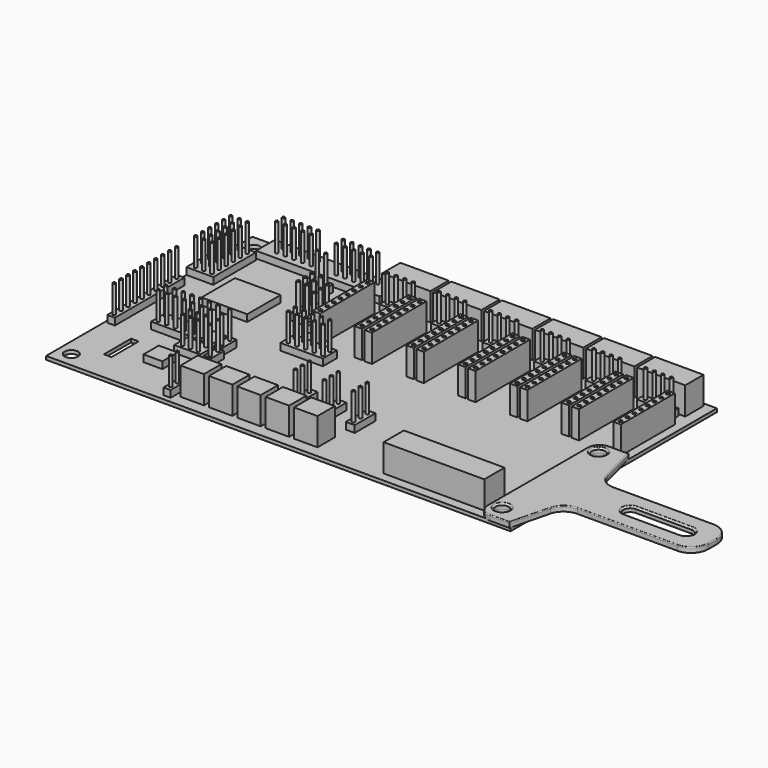
from build123d import *

# Parameters (mm, degrees)
F0_W           = 2.1383463393
F0_H           = 19.7797067453
F0_R           = 0.4865075134
F1_DEPTH       = 8
F0_H_2         = 19.6269687937
F0_R_2         = 1.9460300534
F0_W_2         = 2.2147138911
F0_H_3         = 9.8727391815
F0_W_3         = 5.479511394
F0_H_4         = 5.554471502
F0_W_4         = 2.0619777519
F0_H_5         = 4.9640203219
F0_W_5         = 6.8159792801
F0_H_6         = 6.2813939898
F0_W_6         = 2.5666546012
F0_H_7         = 7.4842127053
F0_W_7         = 7.560583364
F0_H_8         = 4.8876486276
F0_W_8         = 2.1383453036
F0_H_9         = 4.6859326135
F0_W_9         = 17.6604543653
F0_H_10        = 5.1752777491
F0_W_10        = 2.2910845498
F0_H_11        = 25.2068089793
F0_W_11        = 13.2490306353
F0_H_12        = 12.1427537582
F0_W_12        = 12.365488222
F0_H_13        = 5.121120681
F0_W_13        = 2.2910866211
F0_H_14        = 7.1787352486
F0_W_14        = 5.0641262077
F0_H_15        = 7.3660017566
F0_W_15        = 4.9640203219
F0_H_16        = 2.4147640345
F0_R_3         = 1.6205905882
F0_W_16        = 10.0807783365
F0_H_17        = 2.5201944547
F0_W_17        = 14.0519930406
F0_H_18        = 6.6441499584
F2_DEPTH       = 1
F0_W_18        = 7.8297872952
F0_H_19        = 15.5030138078
F0_R_4         = 0.41700644
F0_W_19        = 17.9754786721
F0_H_20        = 6.8159803158
F3_DEPTH       = 2
F3_DEPTH_BACK  = 1
F0_W_20        = 9.8887440656
F0_H_21        = 7.3633516746
F0_W_21        = 9.622558009
F0_W_22        = 9.7573204997
F4_DEPTH       = 8
F4_DEPTH_BACK  = 1
F0_R_5         = 0.5
F5_DEPTH       = 2
F5_DEPTH_BACK  = 1
F6_DEPTH       = 8
F6_DEPTH_BACK  = 1
F7_DEPTH       = 2
F7_DEPTH_BACK  = 1
F8_R           = 2.1799728678
F8_R_2         = 2
F8_R_3         = 2.5
F9_DEPTH       = 4
F10_DEPTH      = 10
F10_DEPTH_BACK = 1
F11_R          = 1.9460300534
F12_DEPTH      = 1.5
F13_SIZE       = 0.5
F14_R          = 0.25


# Not quite as in the source:
# - a feature names something its author has since deleted; it is built from what else it names


with BuildPart() as f1:
    # F0 (on Top) → F1 (new body)
    with BuildSketch(Plane.XY):
        with Locations((5.3948195173, 11.5601837436)):
            Rectangle(F0_W, F0_H)
        with Locations((5.4469605535, 3.0105938525)):
            Circle(F0_R, mode=Mode.SUBTRACT)
        with Locations((5.439511834, 5.4706814883)):
            Circle(F0_R, mode=Mode.SUBTRACT)
        with Locations((5.4320631146, 7.9307691241)):
            Circle(F0_R, mode=Mode.SUBTRACT)
        with Locations((5.4246143951, 10.3908567598)):
            Circle(F0_R, mode=Mode.SUBTRACT)
        with Locations((5.4171656757, 12.8509443956)):
            Circle(F0_R, mode=Mode.SUBTRACT)
        with Locations((5.4097169562, 15.3110320313)):
            Circle(F0_R, mode=Mode.SUBTRACT)
        with Locations((5.4022682368, 17.7711196671)):
            Circle(F0_R, mode=Mode.SUBTRACT)
        with Locations((5.3948195173, 20.2312073029)):
            Circle(F0_R, mode=Mode.SUBTRACT)
    extrude(amount=F1_DEPTH)

    # F8 (on face) → F9 (cut)
    with BuildSketch(Plane.XY.offset(8)):
        with Locations((-23.1175161898, -59.319212369)):
            Circle(F8_R)
        with Locations((-16.9533622074, -59.319212369)):
            Circle(F8_R_2)
        with Locations((-8.2318261898, -59.319212369)):
            Circle(F8_R)
        with Locations((-2.0676722074, -59.319212369)):
            Circle(F8_R_2)
        with Locations((6.6538638102, -59.319212369)):
            Circle(F8_R)
        with Locations((12.8180177926, -59.319212369)):
            Circle(F8_R_2)
        with Locations((21.5395538102, -59.319212369)):
            Circle(F8_R)
        with Locations((27.7037077926, -59.319212369)):
            Circle(F8_R_2)
        with Locations((36.4252438102, -59.319212369)):
            Circle(F8_R)
        with Locations((42.5893977926, -59.319212369)):
            Circle(F8_R_2)
        with Locations((84.719479084, -59.7627162933)):
            Circle(F8_R_3)
        with Locations((93.9138680696, -59.7627162933)):
            Circle(F8_R_3)
        with Locations((102.625829084, -59.7627162933)):
            Circle(F8_R_3)
        with Locations((111.8202180696, -59.7627162933)):
            Circle(F8_R_3)
        with Locations((120.532179084, -59.7627162933)):
            Circle(F8_R_3)
        with Locations((129.7265680696, -59.7627162933)):
            Circle(F8_R_3)
    extrude(amount=-F9_DEPTH, mode=Mode.SUBTRACT)


with BuildPart() as f1b:
    # F0 (on Top) → F1, piece 2 (new body)
    with BuildSketch(Plane.XY):
        with Locations((17.4835866574, 11.560184132)):
            Rectangle(F0_W, F0_H_2)
        with Locations((17.538712812, 3.0105938525)):
            Circle(F0_R, mode=Mode.SUBTRACT)
        with Locations((17.5312640925, 5.4706814883)):
            Circle(F0_R, mode=Mode.SUBTRACT)
        with Locations((17.5238153731, 7.9307691241)):
            Circle(F0_R, mode=Mode.SUBTRACT)
        with Locations((17.5163666537, 10.3908567598)):
            Circle(F0_R, mode=Mode.SUBTRACT)
        with Locations((17.5089179342, 12.8509443956)):
            Circle(F0_R, mode=Mode.SUBTRACT)
        with Locations((17.5014692148, 15.3110320313)):
            Circle(F0_R, mode=Mode.SUBTRACT)
        with Locations((17.4940204953, 17.7711196671)):
            Circle(F0_R, mode=Mode.SUBTRACT)
        with Locations((17.4865717759, 20.2312073029)):
            Circle(F0_R, mode=Mode.SUBTRACT)
    extrude(amount=F1_DEPTH)


with BuildPart() as f1c:
    # F0 (on Top) → F1, piece 3 (new body)
    with BuildSketch(Plane.XY):
        with Locations((20.4430973949, 11.5601837436)):
            Rectangle(F0_W, F0_H)
        with Locations((20.4900175104, 3.0105938525)):
            Circle(F0_R, mode=Mode.SUBTRACT)
        with Locations((20.4825687909, 5.4706814883)):
            Circle(F0_R, mode=Mode.SUBTRACT)
        with Locations((20.4751200715, 7.9307691241)):
            Circle(F0_R, mode=Mode.SUBTRACT)
        with Locations((20.467671352, 10.3908567598)):
            Circle(F0_R, mode=Mode.SUBTRACT)
        with Locations((20.4602226326, 12.8509443956)):
            Circle(F0_R, mode=Mode.SUBTRACT)
        with Locations((20.4527739131, 15.3110320313)):
            Circle(F0_R, mode=Mode.SUBTRACT)
        with Locations((20.4453251937, 17.7711196671)):
            Circle(F0_R, mode=Mode.SUBTRACT)
        with Locations((20.4378764742, 20.2312073029)):
            Circle(F0_R, mode=Mode.SUBTRACT)
    extrude(amount=F1_DEPTH)


with BuildPart() as f1d:
    # F0 (on Top) → F1, piece 4 (new body)
    with BuildSketch(Plane.XY):
        with Locations((32.5318645349, 11.560184132)):
            Rectangle(F0_W, F0_H_2)
        with Locations((32.5817697689, 3.0105938525)):
            Circle(F0_R, mode=Mode.SUBTRACT)
        with Locations((32.5743210495, 5.4706814883)):
            Circle(F0_R, mode=Mode.SUBTRACT)
        with Locations((32.56687233, 7.9307691241)):
            Circle(F0_R, mode=Mode.SUBTRACT)
        with Locations((32.5594236106, 10.3908567598)):
            Circle(F0_R, mode=Mode.SUBTRACT)
        with Locations((32.5519748911, 12.8509443956)):
            Circle(F0_R, mode=Mode.SUBTRACT)
        with Locations((32.5445261717, 15.3110320313)):
            Circle(F0_R, mode=Mode.SUBTRACT)
        with Locations((32.5370774522, 17.7711196671)):
            Circle(F0_R, mode=Mode.SUBTRACT)
        with Locations((32.5296287328, 20.2312073029)):
            Circle(F0_R, mode=Mode.SUBTRACT)
    extrude(amount=F1_DEPTH)


with BuildPart() as f1e:
    # F0 (on Top) → F1, piece 5 (new body)
    with BuildSketch(Plane.XY):
        with Locations((35.4913752724, 11.5601837436)):
            Rectangle(F0_W, F0_H)
        with Locations((35.5330744673, 3.0105938525)):
            Circle(F0_R, mode=Mode.SUBTRACT)
        with Locations((35.5256257478, 5.4706814883)):
            Circle(F0_R, mode=Mode.SUBTRACT)
        with Locations((35.5181770284, 7.9307691241)):
            Circle(F0_R, mode=Mode.SUBTRACT)
        with Locations((35.5107283089, 10.3908567598)):
            Circle(F0_R, mode=Mode.SUBTRACT)
        with Locations((35.5032795895, 12.8509443956)):
            Circle(F0_R, mode=Mode.SUBTRACT)
        with Locations((35.49583087, 15.3110320313)):
            Circle(F0_R, mode=Mode.SUBTRACT)
        with Locations((35.4883821506, 17.7711196671)):
            Circle(F0_R, mode=Mode.SUBTRACT)
        with Locations((35.4809334311, 20.2312073029)):
            Circle(F0_R, mode=Mode.SUBTRACT)
    extrude(amount=F1_DEPTH)


with BuildPart() as f1f:
    # F0 (on Top) → F1, piece 6 (new body)
    with BuildSketch(Plane.XY):
        with Locations((47.5801424125, 11.560184132)):
            Rectangle(F0_W, F0_H_2)
        with Locations((47.6248267258, 3.0105938525)):
            Circle(F0_R, mode=Mode.SUBTRACT)
        with Locations((47.6173780064, 5.4706814883)):
            Circle(F0_R, mode=Mode.SUBTRACT)
        with Locations((47.6099292869, 7.9307691241)):
            Circle(F0_R, mode=Mode.SUBTRACT)
        with Locations((47.6024805675, 10.3908567598)):
            Circle(F0_R, mode=Mode.SUBTRACT)
        with Locations((47.595031848, 12.8509443956)):
            Circle(F0_R, mode=Mode.SUBTRACT)
        with Locations((47.5875831286, 15.3110320313)):
            Circle(F0_R, mode=Mode.SUBTRACT)
        with Locations((47.5801344091, 17.7711196671)):
            Circle(F0_R, mode=Mode.SUBTRACT)
        with Locations((47.5726856897, 20.2312073029)):
            Circle(F0_R, mode=Mode.SUBTRACT)
    extrude(amount=F1_DEPTH)


with BuildPart() as f1g:
    # F0 (on Top) → F1, piece 7 (new body)
    with BuildSketch(Plane.XY):
        with Locations((50.5396531499, 11.5601837436)):
            Rectangle(F0_W, F0_H)
        with Locations((50.5761314242, 3.0105938525)):
            Circle(F0_R, mode=Mode.SUBTRACT)
        with Locations((50.5686827047, 5.4706814883)):
            Circle(F0_R, mode=Mode.SUBTRACT)
        with Locations((50.5612339853, 7.9307691241)):
            Circle(F0_R, mode=Mode.SUBTRACT)
        with Locations((50.5537852658, 10.3908567598)):
            Circle(F0_R, mode=Mode.SUBTRACT)
        with Locations((50.5463365464, 12.8509443956)):
            Circle(F0_R, mode=Mode.SUBTRACT)
        with Locations((50.5388878269, 15.3110320313)):
            Circle(F0_R, mode=Mode.SUBTRACT)
        with Locations((50.5314391075, 17.7711196671)):
            Circle(F0_R, mode=Mode.SUBTRACT)
        with Locations((50.523990388, 20.2312073029)):
            Circle(F0_R, mode=Mode.SUBTRACT)
    extrude(amount=F1_DEPTH)


with BuildPart() as f1h:
    # F0 (on Top) → F1, piece 8 (new body)
    with BuildSketch(Plane.XY):
        with Locations((62.62842029, 11.560184132)):
            Rectangle(F0_W, F0_H_2)
        with Locations((62.6678836827, 3.0105938525)):
            Circle(F0_R, mode=Mode.SUBTRACT)
        with Locations((62.6604349633, 5.4706814883)):
            Circle(F0_R, mode=Mode.SUBTRACT)
        with Locations((62.6529862438, 7.9307691241)):
            Circle(F0_R, mode=Mode.SUBTRACT)
        with Locations((62.6455375244, 10.3908567598)):
            Circle(F0_R, mode=Mode.SUBTRACT)
        with Locations((62.6380888049, 12.8509443956)):
            Circle(F0_R, mode=Mode.SUBTRACT)
        with Locations((62.6306400855, 15.3110320313)):
            Circle(F0_R, mode=Mode.SUBTRACT)
        with Locations((62.623191366, 17.7711196671)):
            Circle(F0_R, mode=Mode.SUBTRACT)
        with Locations((62.6157426466, 20.2312073029)):
            Circle(F0_R, mode=Mode.SUBTRACT)
    extrude(amount=F1_DEPTH)


with BuildPart() as f1i:
    # F0 (on Top) → F1, piece 9 (new body)
    with BuildSketch(Plane.XY):
        with Locations((65.5879310275, 11.5601837436)):
            Rectangle(F0_W, F0_H)
        with Locations((65.6191883811, 3.0105938525)):
            Circle(F0_R, mode=Mode.SUBTRACT)
        with Locations((65.6117396616, 5.4706814883)):
            Circle(F0_R, mode=Mode.SUBTRACT)
        with Locations((65.6042909422, 7.9307691241)):
            Circle(F0_R, mode=Mode.SUBTRACT)
        with Locations((65.5968422228, 10.3908567598)):
            Circle(F0_R, mode=Mode.SUBTRACT)
        with Locations((65.5893935033, 12.8509443956)):
            Circle(F0_R, mode=Mode.SUBTRACT)
        with Locations((65.5819447839, 15.3110320313)):
            Circle(F0_R, mode=Mode.SUBTRACT)
        with Locations((65.5744960644, 17.7711196671)):
            Circle(F0_R, mode=Mode.SUBTRACT)
        with Locations((65.567047345, 20.2312073029)):
            Circle(F0_R, mode=Mode.SUBTRACT)
    extrude(amount=F1_DEPTH)


with BuildPart() as f1j:
    # F0 (on Top) → F1, piece 10 (new body)
    with BuildSketch(Plane.XY):
        with Locations((77.6766981675, 11.560184132)):
            Rectangle(F0_W, F0_H_2)
        with Locations((77.7109406396, 3.0105938525)):
            Circle(F0_R, mode=Mode.SUBTRACT)
        with Locations((77.7034919202, 5.4706814883)):
            Circle(F0_R, mode=Mode.SUBTRACT)
        with Locations((77.6960432007, 7.9307691241)):
            Circle(F0_R, mode=Mode.SUBTRACT)
        with Locations((77.6885944813, 10.3908567598)):
            Circle(F0_R, mode=Mode.SUBTRACT)
        with Locations((77.6811457618, 12.8509443956)):
            Circle(F0_R, mode=Mode.SUBTRACT)
        with Locations((77.6736970424, 15.3110320313)):
            Circle(F0_R, mode=Mode.SUBTRACT)
        with Locations((77.6662483229, 17.7711196671)):
            Circle(F0_R, mode=Mode.SUBTRACT)
        with Locations((77.6587996035, 20.2312073029)):
            Circle(F0_R, mode=Mode.SUBTRACT)
    extrude(amount=F1_DEPTH)


with BuildPart() as f1k:
    # F0 (on Top) → F1, piece 11 (new body)
    with BuildSketch(Plane.XY):
        with Locations((80.636208905, 11.5601837436)):
            Rectangle(F0_W, F0_H)
        with Locations((80.662245338, 3.0105938525)):
            Circle(F0_R, mode=Mode.SUBTRACT)
        with Locations((80.6547966186, 5.4706814883)):
            Circle(F0_R, mode=Mode.SUBTRACT)
        with Locations((80.6473478991, 7.9307691241)):
            Circle(F0_R, mode=Mode.SUBTRACT)
        with Locations((80.6398991797, 10.3908567598)):
            Circle(F0_R, mode=Mode.SUBTRACT)
        with Locations((80.6324504602, 12.8509443956)):
            Circle(F0_R, mode=Mode.SUBTRACT)
        with Locations((80.6250017408, 15.3110320313)):
            Circle(F0_R, mode=Mode.SUBTRACT)
        with Locations((80.6175530213, 17.7711196671)):
            Circle(F0_R, mode=Mode.SUBTRACT)
        with Locations((80.6101043019, 20.2312073029)):
            Circle(F0_R, mode=Mode.SUBTRACT)
    extrude(amount=F1_DEPTH)


with BuildPart() as f1l:
    # F0 (on Top) → F1, piece 12 (new body)
    with BuildSketch(Plane.XY):
        with Locations((92.7249760451, 11.560184132)):
            Rectangle(F0_W, F0_H_2)
        with Locations((92.7539975965, 3.0105938525)):
            Circle(F0_R, mode=Mode.SUBTRACT)
        with Locations((92.7465488771, 5.4706814883)):
            Circle(F0_R, mode=Mode.SUBTRACT)
        with Locations((92.7391001577, 7.9307691241)):
            Circle(F0_R, mode=Mode.SUBTRACT)
        with Locations((92.7316514382, 10.3908567598)):
            Circle(F0_R, mode=Mode.SUBTRACT)
        with Locations((92.7242027188, 12.8509443956)):
            Circle(F0_R, mode=Mode.SUBTRACT)
        with Locations((92.7167539993, 15.3110320313)):
            Circle(F0_R, mode=Mode.SUBTRACT)
        with Locations((92.7093052799, 17.7711196671)):
            Circle(F0_R, mode=Mode.SUBTRACT)
        with Locations((92.7018565604, 20.2312073029)):
            Circle(F0_R, mode=Mode.SUBTRACT)
    extrude(amount=F1_DEPTH)


with BuildPart() as f2:
    # F0 (on Top) → F2 (new body)
    with BuildSketch(Plane.XY):
        Polygon((-38.7532671023, 33.5722392425), (-38.7532671023, 31.7772014981), (-38.7532671023, 25.0439776386), (-30.9234798072, 25.0439776386), (-30.9234798072, 9.5409638307), (-38.7532671023, 9.5409638307), (-38.7532671023, -41.4277607575), (96.2467328977, -41.4277607575), (96.2467328977, 33.5722392425), align=None)
        with Locations((-34.8440401784, -37.1435576593)):
            Circle(F0_R_2, mode=Mode.SUBTRACT)
        with Locations((-27.887346881, -27.6786446647)):
            Rectangle(F0_W_2, F0_H_3, mode=Mode.SUBTRACT)
        with Locations((-16.8053327625, -27.2508614757)):
            Rectangle(F0_W_3, F0_H_4, mode=Mode.SUBTRACT)
        with Locations((-4.8237512626, -37.3881089662)):
            Rectangle(F0_W_4, F0_H_5, mode=Mode.SUBTRACT)
        with Locations((1.0400285531, -34.9124877097)):
            Rectangle(F0_W_5, F0_H_6, mode=Mode.SUBTRACT)
        with Locations((9.2893166707, -34.9124877097)):
            Rectangle(F0_W_5, F0_H_6, mode=Mode.SUBTRACT)
        with Locations((17.5386047883, -34.9124877097)):
            Rectangle(F0_W_5, F0_H_6, mode=Mode.SUBTRACT)
        with Locations((25.7878929059, -34.9124877097)):
            Rectangle(F0_W_5, F0_H_6, mode=Mode.SUBTRACT)
        with Locations((21.5385374591, -23.5010766555)):
            Rectangle(F0_W_6, F0_H_7, mode=Mode.SUBTRACT)
        with Locations((-13.2243989271, -19.6321943845)):
            Rectangle(F0_W_7, F0_H_8, mode=Mode.SUBTRACT)
        with Locations((-7.3821305288, -19.6554254934)):
            Rectangle(F0_W_8, F0_H_9, mode=Mode.SUBTRACT)
        with Locations((-19.4389688494, -13.7994720597)):
            Rectangle(F0_W_9, F0_H_10, mode=Mode.SUBTRACT)
        with Locations((-8.7009054267, -13.773147992)):
            Rectangle(F0_W_10, F0_H_10, mode=Mode.SUBTRACT)
        with Locations((-36.9753206354, -7.4155029606)):
            Rectangle(F0_W_2, F0_H_11, mode=Mode.SUBTRACT)
        with Locations((34.0371810235, -34.9124877097)):
            Rectangle(F0_W_5, F0_H_6, mode=Mode.SUBTRACT)
        with Locations((29.940144129, -23.5010766555)):
            Rectangle(F0_W_6, F0_H_7, mode=Mode.SUBTRACT)
        with Locations((38.3417507989, -23.5010766555)):
            Rectangle(F0_W_6, F0_H_7, mode=Mode.SUBTRACT)
        Polygon((57.1692081971, -38.6863915229), (57.1692081971, -31.3230398483), (67.0579522627, -31.3230398483), (76.6805102716, -31.3230398483), (86.4378307714, -31.3230398483), (86.4378307714, -38.6863915229), (76.6805102716, -38.6863915229), (67.0579522627, -38.6863915229), align=None, mode=Mode.SUBTRACT)
        with Locations((90.3885619373, -37.1455874826)):
            Circle(F0_R_2, mode=Mode.SUBTRACT)
        with Locations((-20.1162074077, 6.1425196168)):
            Rectangle(F0_W_11, F0_H_12, mode=Mode.SUBTRACT)
        with Locations((7.3327940732, -3.6349598129)):
            Rectangle(F0_W_12, F0_H_13, mode=Mode.SUBTRACT)
        with Locations((1.1712568996, 8.2426817919)):
            Rectangle(F0_W_13, F0_H_14, mode=Mode.SUBTRACT)
        with Locations((-3.7398368359, 10.5292772493)):
            Rectangle(F0_W_14, F0_H_15, mode=Mode.SUBTRACT)
        with Locations((5.3948195173, 11.5601837436)):
            Rectangle(F0_W, F0_H, mode=Mode.SUBTRACT)
        with Locations((17.4835866574, 11.560184132)):
            Rectangle(F0_W, F0_H_2, mode=Mode.SUBTRACT)
        with Locations((20.4430973949, 11.5601837436)):
            Rectangle(F0_W, F0_H, mode=Mode.SUBTRACT)
        with Locations((-9.9405092772, 22.5856218906)):
            Rectangle(F0_W_15, F0_H_16, mode=Mode.SUBTRACT)
        with Locations((-34.9667365808, 29.4120077307)):
            Circle(F0_R_3, mode=Mode.SUBTRACT)
        Polygon((-31.4407066232, 25.7186289664), (-31.4407066232, 32.5346092821), (-13.4652279511, 32.5346092821), (4.510250721, 32.5346092821), (4.510250721, 25.7186289664), (-13.4652279511, 25.7186289664), align=None, mode=Mode.SUBTRACT)
        with Locations((11.9188682081, 23.9329783236)):
            Rectangle(F0_W_16, F0_H_17, mode=Mode.SUBTRACT)
        with Locations((26.8882540273, 23.9329783236)):
            Rectangle(F0_W_16, F0_H_17, mode=Mode.SUBTRACT)
        with Locations((12.0708325316, 29.2316274854)):
            Rectangle(F0_W_17, F0_H_18, mode=Mode.SUBTRACT)
        with Locations((26.887482792, 29.2316274854)):
            Rectangle(F0_W_17, F0_H_18, mode=Mode.SUBTRACT)
        with Locations((32.5318645349, 11.560184132)):
            Rectangle(F0_W, F0_H_2, mode=Mode.SUBTRACT)
        with Locations((35.4913752724, 11.5601837436)):
            Rectangle(F0_W, F0_H, mode=Mode.SUBTRACT)
        with Locations((47.5801424125, 11.560184132)):
            Rectangle(F0_W, F0_H_2, mode=Mode.SUBTRACT)
        with Locations((50.5396531499, 11.5601837436)):
            Rectangle(F0_W, F0_H, mode=Mode.SUBTRACT)
        with Locations((90.3885619373, -2.1260819313)):
            Circle(F0_R_2, mode=Mode.SUBTRACT)
        with Locations((62.62842029, 11.560184132)):
            Rectangle(F0_W, F0_H_2, mode=Mode.SUBTRACT)
        with Locations((65.5879310275, 11.5601837436)):
            Rectangle(F0_W, F0_H, mode=Mode.SUBTRACT)
        with Locations((77.6766981675, 11.560184132)):
            Rectangle(F0_W, F0_H_2, mode=Mode.SUBTRACT)
        with Locations((80.636208905, 11.5601837436)):
            Rectangle(F0_W, F0_H, mode=Mode.SUBTRACT)
        with Locations((92.7249760451, 11.560184132)):
            Rectangle(F0_W, F0_H_2, mode=Mode.SUBTRACT)
        with Locations((41.8576398464, 23.9329783236)):
            Rectangle(F0_W_16, F0_H_17, mode=Mode.SUBTRACT)
        with Locations((56.8270256656, 23.9329783236)):
            Rectangle(F0_W_16, F0_H_17, mode=Mode.SUBTRACT)
        with Locations((41.7041330524, 29.2316274854)):
            Rectangle(F0_W_17, F0_H_18, mode=Mode.SUBTRACT)
        with Locations((56.5207833128, 29.2316274854)):
            Rectangle(F0_W_17, F0_H_18, mode=Mode.SUBTRACT)
        with Locations((71.7964114848, 23.9329783236)):
            Rectangle(F0_W_16, F0_H_17, mode=Mode.SUBTRACT)
        with Locations((86.765797304, 23.9329783236)):
            Rectangle(F0_W_16, F0_H_17, mode=Mode.SUBTRACT)
        with Locations((71.3374335732, 29.2316274854)):
            Rectangle(F0_W_17, F0_H_18, mode=Mode.SUBTRACT)
        with Locations((86.1540838336, 29.2316274854)):
            Rectangle(F0_W_17, F0_H_18, mode=Mode.SUBTRACT)
    extrude(amount=-F2_DEPTH)

    # F0 (on Top) → F3 (join, two sides)
    with BuildSketch(Plane.XY) as f3_sk:
        with Locations((-34.8383734548, 17.2924707347)):
            Rectangle(F0_W_18, F0_H_19)
        with Locations((-37.078142586, 10.8069347614)):
            Circle(F0_R_4, mode=Mode.SUBTRACT)
        with Locations((-34.6817455773, 10.8069347614)):
            Circle(F0_R_4, mode=Mode.SUBTRACT)
        with Locations((-32.2853485686, 10.8069347614)):
            Circle(F0_R_4, mode=Mode.SUBTRACT)
        with Locations((-37.0635132799, 13.3533761215)):
            Circle(F0_R_4, mode=Mode.SUBTRACT)
        with Locations((-34.6671162713, 13.3533761215)):
            Circle(F0_R_4, mode=Mode.SUBTRACT)
        with Locations((-32.2707192626, 13.3533761215)):
            Circle(F0_R_4, mode=Mode.SUBTRACT)
        with Locations((-37.0488839739, 15.8998174816)):
            Circle(F0_R_4, mode=Mode.SUBTRACT)
        with Locations((-34.6524869652, 15.8998174816)):
            Circle(F0_R_4, mode=Mode.SUBTRACT)
        with Locations((-32.2560899566, 15.8998174816)):
            Circle(F0_R_4, mode=Mode.SUBTRACT)
        with Locations((-37.0342546679, 18.4462588418)):
            Circle(F0_R_4, mode=Mode.SUBTRACT)
        with Locations((-34.6378576592, 18.4462588418)):
            Circle(F0_R_4, mode=Mode.SUBTRACT)
        with Locations((-32.2414606505, 18.4462588418)):
            Circle(F0_R_4, mode=Mode.SUBTRACT)
        with Locations((-37.0196253619, 20.9927002019)):
            Circle(F0_R_4, mode=Mode.SUBTRACT)
        with Locations((-34.6232283532, 20.9927002019)):
            Circle(F0_R_4, mode=Mode.SUBTRACT)
        with Locations((-32.2268313445, 20.9927002019)):
            Circle(F0_R_4, mode=Mode.SUBTRACT)
        with Locations((-37.0049960558, 23.5391415621)):
            Circle(F0_R_4, mode=Mode.SUBTRACT)
        with Locations((-34.6085990472, 23.5391415621)):
            Circle(F0_R_4, mode=Mode.SUBTRACT)
        with Locations((-32.2122020385, 23.5391415621)):
            Circle(F0_R_4, mode=Mode.SUBTRACT)
        with Locations((-19.4389688494, -13.7994720597)):
            Rectangle(F0_W_9, F0_H_10)
        with Locations((-27.1577291654, -15.2034537075)):
            Circle(F0_R_4, mode=Mode.SUBTRACT)
        with Locations((-24.6314429908, -15.2034537075)):
            Circle(F0_R_4, mode=Mode.SUBTRACT)
        with Locations((-22.1051568161, -15.2034537075)):
            Circle(F0_R_4, mode=Mode.SUBTRACT)
        with Locations((-19.5788706415, -15.2034537075)):
            Circle(F0_R_4, mode=Mode.SUBTRACT)
        with Locations((-17.0525844669, -15.2034537075)):
            Circle(F0_R_4, mode=Mode.SUBTRACT)
        with Locations((-14.5262982923, -15.2034537075)):
            Circle(F0_R_4, mode=Mode.SUBTRACT)
        with Locations((-12.0000121177, -15.2034537075)):
            Circle(F0_R_4, mode=Mode.SUBTRACT)
        with Locations((-27.1577291654, -12.3954904119)):
            Circle(F0_R_4, mode=Mode.SUBTRACT)
        with Locations((-24.6314429908, -12.3954904119)):
            Circle(F0_R_4, mode=Mode.SUBTRACT)
        with Locations((-22.1051568161, -12.3954904119)):
            Circle(F0_R_4, mode=Mode.SUBTRACT)
        with Locations((-19.5788706415, -12.3954904119)):
            Circle(F0_R_4, mode=Mode.SUBTRACT)
        with Locations((-17.0525844669, -12.3954904119)):
            Circle(F0_R_4, mode=Mode.SUBTRACT)
        with Locations((-14.5262982923, -12.3954904119)):
            Circle(F0_R_4, mode=Mode.SUBTRACT)
        with Locations((-12.0000121177, -12.3954904119)):
            Circle(F0_R_4, mode=Mode.SUBTRACT)
        with Locations((-36.9753206354, -7.4155029606)):
            Rectangle(F0_W_2, F0_H_11)
        with Locations((-37.0629606711, -18.8174451744)):
            Circle(F0_R_4, mode=Mode.SUBTRACT)
        with Locations((-37.0629606711, -16.2902419244)):
            Circle(F0_R_4, mode=Mode.SUBTRACT)
        with Locations((-37.0629606711, -13.7630386744)):
            Circle(F0_R_4, mode=Mode.SUBTRACT)
        with Locations((-37.0629606711, -11.2358354244)):
            Circle(F0_R_4, mode=Mode.SUBTRACT)
        with Locations((-37.0629606711, -8.7086321744)):
            Circle(F0_R_4, mode=Mode.SUBTRACT)
        with Locations((-37.0629606711, -6.1814289244)):
            Circle(F0_R_4, mode=Mode.SUBTRACT)
        with Locations((-37.0629606711, -3.6542256744)):
            Circle(F0_R_4, mode=Mode.SUBTRACT)
        with Locations((-37.0629606711, -1.1270224244)):
            Circle(F0_R_4, mode=Mode.SUBTRACT)
        with Locations((-37.0629606711, 1.4001808255)):
            Circle(F0_R_4, mode=Mode.SUBTRACT)
        with Locations((-37.0629606711, 3.9273840755)):
            Circle(F0_R_4, mode=Mode.SUBTRACT)
        with Locations((7.3327940732, -3.6349598129)):
            Rectangle(F0_W_12, F0_H_13)
        with Locations((2.4687983345, -4.8963822812)):
            Circle(F0_R_4, mode=Mode.SUBTRACT)
        with Locations((4.9796886313, -4.8963822812)):
            Circle(F0_R_4, mode=Mode.SUBTRACT)
        with Locations((7.4905789281, -4.8963822812)):
            Circle(F0_R_4, mode=Mode.SUBTRACT)
        with Locations((10.001469225, -4.8963822812)):
            Circle(F0_R_4, mode=Mode.SUBTRACT)
        with Locations((12.5123595218, -4.8963822812)):
            Circle(F0_R_4, mode=Mode.SUBTRACT)
        with Locations((2.4687983345, -2.3735373447)):
            Circle(F0_R_4, mode=Mode.SUBTRACT)
        with Locations((4.9796886313, -2.3735373447)):
            Circle(F0_R_4, mode=Mode.SUBTRACT)
        with Locations((7.4905789281, -2.3735373447)):
            Circle(F0_R_4, mode=Mode.SUBTRACT)
        with Locations((10.001469225, -2.3735373447)):
            Circle(F0_R_4, mode=Mode.SUBTRACT)
        with Locations((12.5123595218, -2.3735373447)):
            Circle(F0_R_4, mode=Mode.SUBTRACT)
        with Locations((-4.477488615, 29.1266191242)):
            Rectangle(F0_W_19, F0_H_20)
        with Locations((-9.8162656838, 27.8998053443)):
            Circle(F0_R_4, mode=Mode.SUBTRACT)
        with Locations((-7.305380947, 27.8998053443)):
            Circle(F0_R_4, mode=Mode.SUBTRACT)
        with Locations((-9.8162656838, 30.3534329042)):
            Circle(F0_R_4, mode=Mode.SUBTRACT)
        with Locations((-7.305380947, 30.3534329042)):
            Circle(F0_R_4, mode=Mode.SUBTRACT)
        with Locations((-4.7944962103, 27.8998053443)):
            Circle(F0_R_4, mode=Mode.SUBTRACT)
        with Locations((-2.2836114735, 27.8998053443)):
            Circle(F0_R_4, mode=Mode.SUBTRACT)
        with Locations((0.2272732632, 27.8998053443)):
            Circle(F0_R_4, mode=Mode.SUBTRACT)
        with Locations((-4.7944962103, 30.3534329042)):
            Circle(F0_R_4, mode=Mode.SUBTRACT)
        with Locations((-2.2836114735, 30.3534329042)):
            Circle(F0_R_4, mode=Mode.SUBTRACT)
        with Locations((0.2272732632, 30.3534329042)):
            Circle(F0_R_4, mode=Mode.SUBTRACT)
        with Locations((-22.4529672871, 29.1266191242)):
            Rectangle(F0_W_19, F0_H_20)
        with Locations((-27.1577291654, 27.8998053443)):
            Circle(F0_R_4, mode=Mode.SUBTRACT)
        with Locations((-24.6468444286, 27.8998053443)):
            Circle(F0_R_4, mode=Mode.SUBTRACT)
        with Locations((-22.1359596919, 27.8998053443)):
            Circle(F0_R_4, mode=Mode.SUBTRACT)
        with Locations((-27.1577291654, 30.3534329042)):
            Circle(F0_R_4, mode=Mode.SUBTRACT)
        with Locations((-24.6468444286, 30.3534329042)):
            Circle(F0_R_4, mode=Mode.SUBTRACT)
        with Locations((-22.1359596919, 30.3534329042)):
            Circle(F0_R_4, mode=Mode.SUBTRACT)
        with Locations((-19.6250749551, 27.8998053443)):
            Circle(F0_R_4, mode=Mode.SUBTRACT)
        with Locations((-17.1141902183, 27.8998053443)):
            Circle(F0_R_4, mode=Mode.SUBTRACT)
        with Locations((-19.6250749551, 30.3534329042)):
            Circle(F0_R_4, mode=Mode.SUBTRACT)
        with Locations((-17.1141902183, 30.3534329042)):
            Circle(F0_R_4, mode=Mode.SUBTRACT)
        with Locations((-13.2243989271, -19.6321943845)):
            Rectangle(F0_W_7, F0_H_8)
        with Locations((-15.388107186, -21.0129674962)):
            Circle(F0_R_4, mode=Mode.SUBTRACT)
        with Locations((-15.3833877763, -18.2569658673)):
            Circle(F0_R_4, mode=Mode.SUBTRACT)
        with Locations((-13.0997894265, -21.0208046037)):
            Circle(F0_R_4, mode=Mode.SUBTRACT)
        with Locations((-10.8114716671, -21.0286417113)):
            Circle(F0_R_4, mode=Mode.SUBTRACT)
        with Locations((-13.0950565966, -18.2569658673)):
            Circle(F0_R_4, mode=Mode.SUBTRACT)
        with Locations((-10.8067254168, -18.2569658673)):
            Circle(F0_R_4, mode=Mode.SUBTRACT)
        with Locations((-8.7009054267, -13.773147992)):
            Rectangle(F0_W_10, F0_H_10)
        with Locations((-8.6133156073, -15.2726349533)):
            Circle(F0_R_4, mode=Mode.SUBTRACT)
        with Locations((-8.6133156073, -12.3263091661)):
            Circle(F0_R_4, mode=Mode.SUBTRACT)
        with Locations((-7.3821305288, -19.6554254934)):
            Rectangle(F0_W_8, F0_H_9)
        with Locations((-7.3456632234, -21.0881018446)):
            Circle(F0_R_4, mode=Mode.SUBTRACT)
        with Locations((-7.3407336591, -18.2093758303)):
            Circle(F0_R_4, mode=Mode.SUBTRACT)
        with Locations((21.5385374591, -23.5010766555)):
            Rectangle(F0_W_6, F0_H_7)
        with Locations((21.5385374591, -26.1619748775)):
            Circle(F0_R_4, mode=Mode.SUBTRACT)
        with Locations((21.5385374591, -23.6364721534)):
            Circle(F0_R_4, mode=Mode.SUBTRACT)
        with Locations((21.5385374591, -21.1109694293)):
            Circle(F0_R_4, mode=Mode.SUBTRACT)
        with Locations((29.940144129, -23.5010766555)):
            Rectangle(F0_W_6, F0_H_7)
        with Locations((29.967666554, -26.1619748775)):
            Circle(F0_R_4, mode=Mode.SUBTRACT)
        with Locations((29.967666554, -23.6364721534)):
            Circle(F0_R_4, mode=Mode.SUBTRACT)
        with Locations((29.967666554, -21.1109694293)):
            Circle(F0_R_4, mode=Mode.SUBTRACT)
        with Locations((38.3417507989, -23.5010766555)):
            Rectangle(F0_W_6, F0_H_7)
        with Locations((38.396795649, -26.1619748775)):
            Circle(F0_R_4, mode=Mode.SUBTRACT)
        with Locations((38.396795649, -23.6364721534)):
            Circle(F0_R_4, mode=Mode.SUBTRACT)
        with Locations((38.396795649, -21.1109694293)):
            Circle(F0_R_4, mode=Mode.SUBTRACT)
        with Locations((1.1712568996, 8.2426817919)):
            Rectangle(F0_W_13, F0_H_14)
        with Locations((1.2465005685, 5.9075458529)):
            Circle(F0_R_4, mode=Mode.SUBTRACT)
        with Locations((1.1970410359, 8.3272582836)):
            Circle(F0_R_4, mode=Mode.SUBTRACT)
        with Locations((1.1475815032, 10.7469707143)):
            Circle(F0_R_4, mode=Mode.SUBTRACT)
        with Locations((-9.9405092772, 22.5856218906)):
            Rectangle(F0_W_15, F0_H_16)
        with Locations((-11.1332718633, 22.5783286241)):
            Circle(F0_R_4, mode=Mode.SUBTRACT)
        with Locations((-8.662869902, 22.5856218906)):
            Circle(F0_R_4, mode=Mode.SUBTRACT)
    extrude(amount=F3_DEPTH)
    extrude(f3_sk.sketch, amount=-F3_DEPTH_BACK)

    # F0 (on Top) → F4 (join, two sides)
    with BuildSketch(Plane.XY) as f4_sk:
        with Locations((1.0400285531, -34.9124877097)):
            Rectangle(F0_W_5, F0_H_6)
        with Locations((9.2893166707, -34.9124877097)):
            Rectangle(F0_W_5, F0_H_6)
        with Locations((17.5386047883, -34.9124877097)):
            Rectangle(F0_W_5, F0_H_6)
        with Locations((25.7878929059, -34.9124877097)):
            Rectangle(F0_W_5, F0_H_6)
        with Locations((34.0371810235, -34.9124877097)):
            Rectangle(F0_W_5, F0_H_6)
        with Locations((62.1135802299, -35.0047156856)):
            Rectangle(F0_W_20, F0_H_21)
        with Locations((71.8692312672, -35.0047156856)):
            Rectangle(F0_W_21, F0_H_21)
        with Locations((81.5591705215, -35.0047156856)):
            Rectangle(F0_W_22, F0_H_21)
    extrude(amount=F4_DEPTH)
    extrude(f4_sk.sketch, amount=-F4_DEPTH_BACK)

    # F0 (on Top) → F5 (join, two sides)
    with BuildSketch(Plane.XY) as f5_sk:
        with Locations((-20.1162074077, 6.1425196168)):
            Rectangle(F0_W_11, F0_H_12)
        with Locations((-16.8053327625, -27.2508614757)):
            Rectangle(F0_W_3, F0_H_4)
        with Locations((-4.8237512626, -37.3881089662)):
            Rectangle(F0_W_4, F0_H_5)
        with Locations((-4.8578898025, -38.4480146514)):
            Circle(F0_R_4, mode=Mode.SUBTRACT)
        with Locations((-4.8578898025, -36.1329880213)):
            Circle(F0_R_4, mode=Mode.SUBTRACT)
        with Locations((-3.7398368359, 10.5292772493)):
            Rectangle(F0_W_14, F0_H_15)
        with Locations((-4.97369, 8.0287387224)):
            Circle(F0_R_5, mode=Mode.SUBTRACT)
        with Locations((-2.48103, 8.0287387224)):
            Circle(F0_R_5, mode=Mode.SUBTRACT)
        with Locations((-4.97369, 10.54581)):
            Circle(F0_R_5, mode=Mode.SUBTRACT)
        with Locations((-2.48103, 10.54581)):
            Circle(F0_R_5, mode=Mode.SUBTRACT)
        with Locations((-4.97369, 13.0628812776)):
            Circle(F0_R_5, mode=Mode.SUBTRACT)
        with Locations((-2.48103, 13.0628812776)):
            Circle(F0_R_5, mode=Mode.SUBTRACT)
    extrude(amount=F5_DEPTH)
    extrude(f5_sk.sketch, amount=-F5_DEPTH_BACK)

    # F0 (on Top) → F7 (join, two sides)
    with BuildSketch(Plane.XY) as f7_sk:
        with Locations((11.9188682081, 23.9329783236)):
            Rectangle(F0_W_16, F0_H_17)
        with Locations((8.1673537819, 23.9537855014)):
            Circle(F0_R_4, mode=Mode.SUBTRACT)
        with Locations((10.6734790852, 23.9537855014)):
            Circle(F0_R_4, mode=Mode.SUBTRACT)
        with Locations((13.1796043884, 23.9537855014)):
            Circle(F0_R_4, mode=Mode.SUBTRACT)
        with Locations((15.6857296917, 23.9537855014)):
            Circle(F0_R_4, mode=Mode.SUBTRACT)
        with Locations((26.8882540273, 23.9329783236)):
            Rectangle(F0_W_16, F0_H_17)
        with Locations((23.1759437666, 23.9537855014)):
            Circle(F0_R_4, mode=Mode.SUBTRACT)
        with Locations((25.6820690698, 23.9537855014)):
            Circle(F0_R_4, mode=Mode.SUBTRACT)
        with Locations((28.1881943731, 23.9537855014)):
            Circle(F0_R_4, mode=Mode.SUBTRACT)
        with Locations((30.6943196763, 23.9537855014)):
            Circle(F0_R_4, mode=Mode.SUBTRACT)
        with Locations((41.8576398464, 23.9329783236)):
            Rectangle(F0_W_16, F0_H_17)
        with Locations((38.1845337512, 23.9537855014)):
            Circle(F0_R_4, mode=Mode.SUBTRACT)
        with Locations((40.6906590544, 23.9537855014)):
            Circle(F0_R_4, mode=Mode.SUBTRACT)
        with Locations((43.1967843577, 23.9537855014)):
            Circle(F0_R_4, mode=Mode.SUBTRACT)
        with Locations((45.7029096609, 23.9537855014)):
            Circle(F0_R_4, mode=Mode.SUBTRACT)
        with Locations((56.8270256656, 23.9329783236)):
            Rectangle(F0_W_16, F0_H_17)
        with Locations((53.1931237358, 23.9537855014)):
            Circle(F0_R_4, mode=Mode.SUBTRACT)
        with Locations((55.699249039, 23.9537855014)):
            Circle(F0_R_4, mode=Mode.SUBTRACT)
        with Locations((58.2053743423, 23.9537855014)):
            Circle(F0_R_4, mode=Mode.SUBTRACT)
        with Locations((60.7114996456, 23.9537855014)):
            Circle(F0_R_4, mode=Mode.SUBTRACT)
        with Locations((71.7964114848, 23.9329783236)):
            Rectangle(F0_W_16, F0_H_17)
        with Locations((68.2017137204, 23.9537855014)):
            Circle(F0_R_4, mode=Mode.SUBTRACT)
        with Locations((70.7078390237, 23.9537855014)):
            Circle(F0_R_4, mode=Mode.SUBTRACT)
        with Locations((73.2139643269, 23.9537855014)):
            Circle(F0_R_4, mode=Mode.SUBTRACT)
        with Locations((75.7200896302, 23.9537855014)):
            Circle(F0_R_4, mode=Mode.SUBTRACT)
        with Locations((86.765797304, 23.9329783236)):
            Rectangle(F0_W_16, F0_H_17)
        with Locations((83.210303705, 23.9537855014)):
            Circle(F0_R_4, mode=Mode.SUBTRACT)
        with Locations((85.7164290083, 23.9537855014)):
            Circle(F0_R_4, mode=Mode.SUBTRACT)
        with Locations((88.2225543115, 23.9537855014)):
            Circle(F0_R_4, mode=Mode.SUBTRACT)
        with Locations((90.7286796148, 23.9537855014)):
            Circle(F0_R_4, mode=Mode.SUBTRACT)
    extrude(amount=F7_DEPTH)
    extrude(f7_sk.sketch, amount=-F7_DEPTH_BACK)

    # F0 (on Top) → F10 (join, two sides)
    with BuildSketch(Plane.XY) as f10_sk:
        with Locations((-32.2853485686, 10.8069347614)):
            Circle(F0_R_4)
        with Locations((-34.6817455773, 10.8069347614)):
            Circle(F0_R_4)
        with Locations((-37.078142586, 10.8069347614)):
            Circle(F0_R_4)
        with Locations((-37.0635132799, 13.3533761215)):
            Circle(F0_R_4)
        with Locations((-34.6671162713, 13.3533761215)):
            Circle(F0_R_4)
        with Locations((-32.2707192626, 13.3533761215)):
            Circle(F0_R_4)
        with Locations((-32.2560899566, 15.8998174816)):
            Circle(F0_R_4)
        with Locations((-34.6524869652, 15.8998174816)):
            Circle(F0_R_4)
        with Locations((-37.0488839739, 15.8998174816)):
            Circle(F0_R_4)
        with Locations((-32.2414606505, 18.4462588418)):
            Circle(F0_R_4)
        with Locations((-32.2268313445, 20.9927002019)):
            Circle(F0_R_4)
        with Locations((-34.6232283532, 20.9927002019)):
            Circle(F0_R_4)
        with Locations((-34.6378576592, 18.4462588418)):
            Circle(F0_R_4)
        with Locations((-37.0342546679, 18.4462588418)):
            Circle(F0_R_4)
        with Locations((-37.0196253619, 20.9927002019)):
            Circle(F0_R_4)
        with Locations((-37.0049960558, 23.5391415621)):
            Circle(F0_R_4)
        with Locations((-34.6085990472, 23.5391415621)):
            Circle(F0_R_4)
        with Locations((-32.2122020385, 23.5391415621)):
            Circle(F0_R_4)
        with Locations((-12.0000121177, -12.3954904119)):
            Circle(F0_R_4)
        with Locations((-8.6133156073, -12.3263091661)):
            Circle(F0_R_4)
        with Locations((-8.6133156073, -15.2726349533)):
            Circle(F0_R_4)
        with Locations((-12.0000121177, -15.2034537075)):
            Circle(F0_R_4)
        with Locations((-7.3407336591, -18.2093758303)):
            Circle(F0_R_4)
        with Locations((-7.3456632234, -21.0881018446)):
            Circle(F0_R_4)
        with Locations((-10.8067254168, -18.2569658673)):
            Circle(F0_R_4)
        with Locations((-10.8114716671, -21.0286417113)):
            Circle(F0_R_4)
        with Locations((-13.0950565966, -18.2569658673)):
            Circle(F0_R_4)
        with Locations((-13.0997894265, -21.0208046037)):
            Circle(F0_R_4)
        with Locations((-15.3833877763, -18.2569658673)):
            Circle(F0_R_4)
        with Locations((-15.388107186, -21.0129674962)):
            Circle(F0_R_4)
        with Locations((-14.5262982923, -12.3954904119)):
            Circle(F0_R_4)
        with Locations((-14.5262982923, -15.2034537075)):
            Circle(F0_R_4)
        with Locations((-17.0525844669, -15.2034537075)):
            Circle(F0_R_4)
        with Locations((-17.0525844669, -12.3954904119)):
            Circle(F0_R_4)
        with Locations((-19.5788706415, -12.3954904119)):
            Circle(F0_R_4)
        with Locations((-19.5788706415, -15.2034537075)):
            Circle(F0_R_4)
        with Locations((-22.1051568161, -12.3954904119)):
            Circle(F0_R_4)
        with Locations((-22.1051568161, -15.2034537075)):
            Circle(F0_R_4)
        with Locations((-24.6314429908, -12.3954904119)):
            Circle(F0_R_4)
        with Locations((-24.6314429908, -15.2034537075)):
            Circle(F0_R_4)
        with Locations((-27.1577291654, -12.3954904119)):
            Circle(F0_R_4)
        with Locations((-27.1577291654, -15.2034537075)):
            Circle(F0_R_4)
        with Locations((-37.0629606711, -18.8174451744)):
            Circle(F0_R_4)
        with Locations((-37.0629606711, -16.2902419244)):
            Circle(F0_R_4)
        with Locations((-37.0629606711, -13.7630386744)):
            Circle(F0_R_4)
        with Locations((-37.0629606711, -11.2358354244)):
            Circle(F0_R_4)
        with Locations((-37.0629606711, -8.7086321744)):
            Circle(F0_R_4)
        with Locations((-37.0629606711, -6.1814289244)):
            Circle(F0_R_4)
        with Locations((-37.0629606711, -3.6542256744)):
            Circle(F0_R_4)
        with Locations((-37.0629606711, -1.1270224244)):
            Circle(F0_R_4)
        with Locations((-37.0629606711, 3.9273840755)):
            Circle(F0_R_4)
        with Locations((-37.0629606711, 1.4001808255)):
            Circle(F0_R_4)
        with Locations((21.5385374591, -21.1109694293)):
            Circle(F0_R_4)
        with Locations((21.5385374591, -23.6364721534)):
            Circle(F0_R_4)
        with Locations((21.5385374591, -26.1619748775)):
            Circle(F0_R_4)
        with Locations((29.967666554, -21.1109694293)):
            Circle(F0_R_4)
        with Locations((29.967666554, -23.6364721534)):
            Circle(F0_R_4)
        with Locations((29.967666554, -26.1619748775)):
            Circle(F0_R_4)
        with Locations((38.396795649, -21.1109694293)):
            Circle(F0_R_4)
        with Locations((38.396795649, -23.6364721534)):
            Circle(F0_R_4)
        with Locations((38.396795649, -26.1619748775)):
            Circle(F0_R_4)
        with Locations((12.5123595218, -2.3735373447)):
            Circle(F0_R_4)
        with Locations((12.5123595218, -4.8963822812)):
            Circle(F0_R_4)
        with Locations((10.001469225, -2.3735373447)):
            Circle(F0_R_4)
        with Locations((10.001469225, -4.8963822812)):
            Circle(F0_R_4)
        with Locations((7.4905789281, -2.3735373447)):
            Circle(F0_R_4)
        with Locations((7.4905789281, -4.8963822812)):
            Circle(F0_R_4)
        with Locations((4.9796886313, -2.3735373447)):
            Circle(F0_R_4)
        with Locations((4.9796886313, -4.8963822812)):
            Circle(F0_R_4)
        with Locations((2.4687983345, -2.3735373447)):
            Circle(F0_R_4)
        with Locations((2.4687983345, -4.8963822812)):
            Circle(F0_R_4)
        with Locations((1.1475815032, 10.7469707143)):
            Circle(F0_R_4)
        with Locations((1.1970410359, 8.3272582836)):
            Circle(F0_R_4)
        with Locations((1.2465005685, 5.9075458529)):
            Circle(F0_R_4)
        with Locations((0.2272732632, 30.3534329042)):
            Circle(F0_R_4)
        with Locations((0.2272732632, 27.8998053443)):
            Circle(F0_R_4)
        with Locations((-2.2836114735, 30.3534329042)):
            Circle(F0_R_4)
        with Locations((-2.2836114735, 27.8998053443)):
            Circle(F0_R_4)
        with Locations((-4.7944962103, 30.3534329042)):
            Circle(F0_R_4)
        with Locations((-4.7944962103, 27.8998053443)):
            Circle(F0_R_4)
        with Locations((-7.305380947, 30.3534329042)):
            Circle(F0_R_4)
        with Locations((-7.305380947, 27.8998053443)):
            Circle(F0_R_4)
        with Locations((-9.8162656838, 30.3534329042)):
            Circle(F0_R_4)
        with Locations((-9.8162656838, 27.8998053443)):
            Circle(F0_R_4)
        with Locations((-17.1141902183, 30.3534329042)):
            Circle(F0_R_4)
        with Locations((-17.1141902183, 27.8998053443)):
            Circle(F0_R_4)
        with Locations((-19.6250749551, 30.3534329042)):
            Circle(F0_R_4)
        with Locations((-19.6250749551, 27.8998053443)):
            Circle(F0_R_4)
        with Locations((-22.1359596919, 30.3534329042)):
            Circle(F0_R_4)
        with Locations((-22.1359596919, 27.8998053443)):
            Circle(F0_R_4)
        with Locations((-24.6468444286, 30.3534329042)):
            Circle(F0_R_4)
        with Locations((-24.6468444286, 27.8998053443)):
            Circle(F0_R_4)
        with Locations((-27.1577291654, 30.3534329042)):
            Circle(F0_R_4)
        with Locations((-27.1577291654, 27.8998053443)):
            Circle(F0_R_4)
        with Locations((8.1673537819, 23.9537855014)):
            Circle(F0_R_4)
        with Locations((10.6734790852, 23.9537855014)):
            Circle(F0_R_4)
        with Locations((13.1796043884, 23.9537855014)):
            Circle(F0_R_4)
        with Locations((15.6857296917, 23.9537855014)):
            Circle(F0_R_4)
        with Locations((23.1759437666, 23.9537855014)):
            Circle(F0_R_4)
        with Locations((25.6820690698, 23.9537855014)):
            Circle(F0_R_4)
        with Locations((28.1881943731, 23.9537855014)):
            Circle(F0_R_4)
        with Locations((30.6943196763, 23.9537855014)):
            Circle(F0_R_4)
        with Locations((45.7029096609, 23.9537855014)):
            Circle(F0_R_4)
        with Locations((43.1967843577, 23.9537855014)):
            Circle(F0_R_4)
        with Locations((53.1931237358, 23.9537855014)):
            Circle(F0_R_4)
        with Locations((55.699249039, 23.9537855014)):
            Circle(F0_R_4)
        with Locations((58.2053743423, 23.9537855014)):
            Circle(F0_R_4)
        with Locations((60.7114996456, 23.9537855014)):
            Circle(F0_R_4)
        with Locations((40.6906590544, 23.9537855014)):
            Circle(F0_R_4)
        with Locations((38.1845337512, 23.9537855014)):
            Circle(F0_R_4)
        with Locations((68.2017137204, 23.9537855014)):
            Circle(F0_R_4)
        with Locations((70.7078390237, 23.9537855014)):
            Circle(F0_R_4)
        with Locations((73.2139643269, 23.9537855014)):
            Circle(F0_R_4)
        with Locations((75.7200896302, 23.9537855014)):
            Circle(F0_R_4)
        with Locations((83.210303705, 23.9537855014)):
            Circle(F0_R_4)
        with Locations((85.7164290083, 23.9537855014)):
            Circle(F0_R_4)
        with Locations((88.2225543115, 23.9537855014)):
            Circle(F0_R_4)
        with Locations((90.7286796148, 23.9537855014)):
            Circle(F0_R_4)
        with Locations((-11.1332718633, 22.5783286241)):
            Circle(F0_R_4)
        with Locations((-8.662869902, 22.5856218906)):
            Circle(F0_R_4)
        with Locations((-4.8578898025, -36.1329880213)):
            Circle(F0_R_4)
        with Locations((-4.8578898025, -38.4480146514)):
            Circle(F0_R_4)
        with Locations((-2.48103, 13.0628812776)):
            Circle(F0_R_5)
        with Locations((-2.48103, 10.54581)):
            Circle(F0_R_5)
        with Locations((-2.48103, 8.0287387224)):
            Circle(F0_R_5)
        with Locations((-4.97369, 8.0287387224)):
            Circle(F0_R_5)
        with Locations((-4.97369, 10.54581)):
            Circle(F0_R_5)
        with Locations((-4.97369, 13.0628812776)):
            Circle(F0_R_5)
    extrude(amount=F10_DEPTH)
    extrude(f10_sk.sketch, amount=-F10_DEPTH_BACK)


with BuildPart() as f6:
    # F0 (on Top) → F6 (new body, two sides)
    with BuildSketch(Plane.XY) as f6_sk:
        with Locations((12.0708325316, 29.2316274854)):
            Rectangle(F0_W_17, F0_H_18)
    extrude(amount=F6_DEPTH)
    extrude(f6_sk.sketch, amount=-F6_DEPTH_BACK)


with BuildPart() as f6b:
    # F0 (on Top) → F6, piece 2 (new body, two sides)
    with BuildSketch(Plane.XY) as f6_2_sk:
        with Locations((26.887482792, 29.2316274854)):
            Rectangle(F0_W_17, F0_H_18)
    extrude(amount=F6_DEPTH)
    extrude(f6_2_sk.sketch, amount=-F6_DEPTH_BACK)


with BuildPart() as f6c:
    # F0 (on Top) → F6, piece 3 (new body, two sides)
    with BuildSketch(Plane.XY) as f6_3_sk:
        with Locations((41.7041330524, 29.2316274854)):
            Rectangle(F0_W_17, F0_H_18)
    extrude(amount=F6_DEPTH)
    extrude(f6_3_sk.sketch, amount=-F6_DEPTH_BACK)


with BuildPart() as f6d:
    # F0 (on Top) → F6, piece 4 (new body, two sides)
    with BuildSketch(Plane.XY) as f6_4_sk:
        with Locations((56.5207833128, 29.2316274854)):
            Rectangle(F0_W_17, F0_H_18)
    extrude(amount=F6_DEPTH)
    extrude(f6_4_sk.sketch, amount=-F6_DEPTH_BACK)


with BuildPart() as f6e:
    # F0 (on Top) → F6, piece 5 (new body, two sides)
    with BuildSketch(Plane.XY) as f6_5_sk:
        with Locations((71.3374335732, 29.2316274854)):
            Rectangle(F0_W_17, F0_H_18)
    extrude(amount=F6_DEPTH)
    extrude(f6_5_sk.sketch, amount=-F6_DEPTH_BACK)


with BuildPart() as f6f:
    # F0 (on Top) → F6, piece 6 (new body, two sides)
    with BuildSketch(Plane.XY) as f6_6_sk:
        with Locations((86.1540838336, 29.2316274854)):
            Rectangle(F0_W_17, F0_H_18)
    extrude(amount=F6_DEPTH)
    extrude(f6_6_sk.sketch, amount=-F6_DEPTH_BACK)


with BuildPart() as f12:
    # F11 (on face) → F12 (new body)
    with BuildSketch(Plane.XY):
        with BuildLine():
            Line((99.0857406079, -9.7466430456), (96.2467328977, 1.5196985754))
            Line((96.2467328977, 1.5196985754), (96.2467328977, -41.4277607575))
            Line((96.2467328977, -41.4277607575), (89.0421301206, -41.4277607575))
            ThreePointArc((89.0421301206, -41.4277607575), (89.791670473, -41.6943170123), (90.5820432901, -41.784726009))
            Line((90.5820432901, -41.784726009), (96.2467328977, -41.784726009))
            Line((96.2467328977, -41.784726009), (99.0857406079, -30.5183843881))
            ThreePointArc((99.0857406079, -30.5183843881), (100.8608037688, -27.7962361628), (103.9341741678, -26.7401421443))
            Line((103.9341741678, -26.7401421443), (132.9979625344, -26.7401421443))
            ThreePointArc((132.9979625344, -26.7401421443), (136.5334964404, -25.2756760502), (137.9979625344, -21.7401421443))
            Line((137.9979625344, -21.7401421443), (137.9979625344, -18.5248852894))
            ThreePointArc((137.9979625344, -18.5248852894), (136.5334964404, -14.9893513834), (132.9979625344, -13.5248852894))
            Line((132.9979625344, -13.5248852894), (103.9341741678, -13.5248852894))
            ThreePointArc((103.9341741678, -13.5248852894), (100.8608037688, -12.4687912708), (99.0857406079, -9.7466430456))
        make_face()
        with BuildLine():
            ThreePointArc((114.0344366431, -22.1325137168), (112.0344366431, -20.1325137168), (114.0344366431, -18.1325137168))
            Line((114.0344366431, -18.1325137168), (130.3022950888, -18.1325137168))
            ThreePointArc((130.3022950888, -18.1325137168), (132.3022950888, -20.1325137168), (130.3022950888, -22.1325137168))
            Line((130.3022950888, -22.1325137168), (114.0344366431, -22.1325137168))
        make_face(mode=Mode.SUBTRACT)
        with BuildLine():
            Line((96.2467328977, 1.5196985754), (90.5820432901, 1.5196985754))
            ThreePointArc((90.5820432901, 1.5196985754), (88.107169556, 0.4945723095), (87.0820432901, -1.9803014246))
            Line((87.0820432901, -1.9803014246), (87.0820432901, -38.284726009))
            ThreePointArc((87.0820432901, -38.284726009), (87.6122203919, -40.1367929498), (89.0421301206, -41.4277607575))
            Line((89.0421301206, -41.4277607575), (96.2467328977, -41.4277607575))
            Line((96.2467328977, -41.4277607575), (96.2467328977, 1.5196985754))
        make_face()
        with Locations((90.3885619373, -37.1455874826)):
            Circle(F11_R, mode=Mode.SUBTRACT)
        with Locations((90.3885619373, -2.1260819313)):
            Circle(F11_R, mode=Mode.SUBTRACT)
    extrude(amount=F12_DEPTH)

    # F13
    f13_edges = [f12.edges().sort_by_distance(p)[0] for p in [
        (88.442532, -2.126082, 1.5),
        (88.442532, -37.145587, 1.5),
        (132.302295, -20.132514, 1.5),
    ]]
    chamfer(f13_edges, length=F13_SIZE)

    # F14
    f14_edges = [f12.edges().sort_by_distance(p)[0] for p in [
        (87.942532, -2.126082, 1.5),
        (136.533496, -25.275676, 1.5),
        (137.997963, -20.132514, 1.5),
        (136.533496, -14.989351, 1.5),
        (118.466068, -13.524885, 1.5),
        (100.860804, -12.468791, 1.5),
        (97.666237, -4.113472, 1.5),
        (93.414388, 1.519699, 1.5),
        (88.10717, 0.494572, 1.5),
        (87.082043, -20.132514, 1.5),
        (88.10717, -40.7596, 1.5),
        (93.414388, -41.784726, 1.5),
        (97.666237, -36.151555, 1.5),
        (100.860804, -27.796236, 1.5),
        (118.466068, -26.740142, 1.5),
        (87.942532, -37.145587, 1.5),
        (132.802295, -20.132514, 1.5),
        (122.168366, -17.632514, 1.5),
        (122.168366, -22.632514, 1.5),
        (111.534437, -20.132514, 1.5),
    ]]
    fillet(f14_edges, radius=F14_R)


solid = Compound([f1.part, f1b.part, f1c.part, f1d.part, f1e.part, f1f.part, f1g.part, f1h.part, f1i.part, f1j.part, f1k.part, f1l.part, f2.part, f6.part, f6b.part, f6c.part, f6d.part, f6e.part, f6f.part, f12.part])
